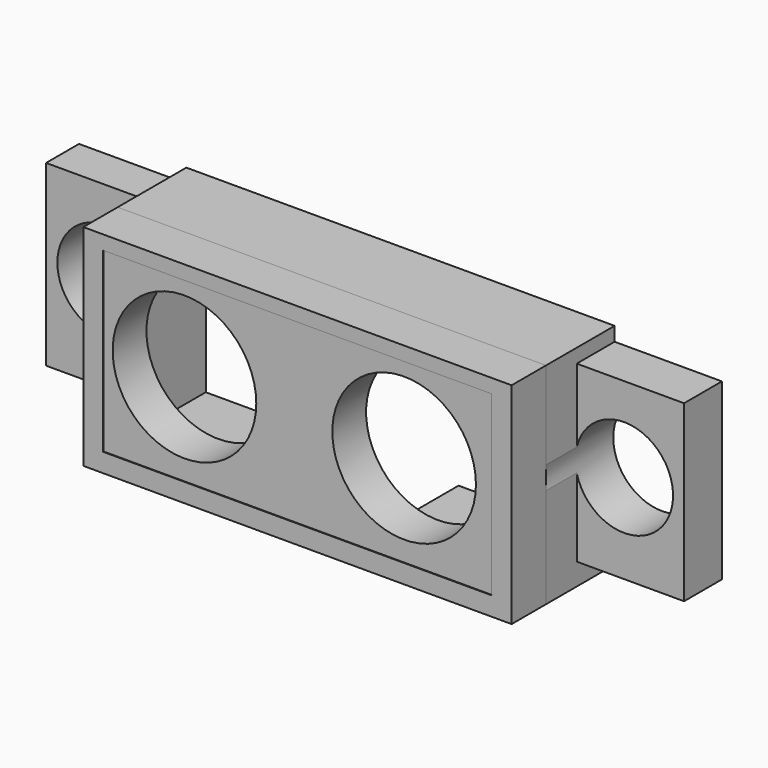
from build123d import *

# Parameters (mm, degrees)
F0_W      = 46
F0_H      = 21
F0_R      = 8.5
F1_DEPTH  = 5
F2_W      = 50.6975790486
F2_H      = 24.8879023129
F2_W_2    = 46
F2_H_2    = 21
F3_DEPTH  = 25.4
F4_W      = 14.5150721073
F4_H      = 25.4
F5_DEPTH  = 14.732
F6_W      = 50.6975790486
F6_H      = 24.8879023129
F7_DEPTH  = 10.16
F8_W      = 14.5150721073
F8_H      = 2.2287086546
F9_DEPTH  = 5.08
F10_DEPTH = 7.874
F12_W     = 2.0801138837
F12_H     = 21.1301185191
F14_DEPTH = 12.7
F13_W     = 2.8098069835
F13_H     = 20.6354465336
F15_DEPTH = 12.7
F16_DEPTH = 2.794
F17_R     = 5.7785
F18_DEPTH = 25.4


# Not quite as in the source:
# - a feature of the source that left no trace in its solid (it failed there, or was rolled back) is left out


with BuildPart() as f1:
    # F0 (on Front) → F1 (new body)
    with BuildSketch(Plane.XZ):
        with Locations((-23, -10.5)):
            Rectangle(F0_W, F0_H)
        with Locations((-36.3915145417, -10.1194066999)):
            Circle(F0_R, mode=Mode.SUBTRACT)
        with Locations((-10.3915145417, -10.1194066999)):
            Circle(F0_R, mode=Mode.SUBTRACT)
    extrude(amount=F1_DEPTH)


with BuildPart() as f3:
    # F2 (on face) → F3 (new body)
    with BuildSketch(Plane(origin=(0, 0, 0), x_dir=(-1, 0, 0), z_dir=(0, 1, 0))):
        with Locations((22.9521770962, -10.7847574982)):
            Rectangle(F2_W, F2_H)
        with Locations((23, -10.5)):
            Rectangle(F2_W_2, F2_H_2, mode=Mode.SUBTRACT)
    extrude(amount=F3_DEPTH)

    # F4 (on face) → F5 (cut)
    with BuildSketch(Plane.XY.offset(-21)):
        with Locations((-23.3345888555, 12.7)):
            Rectangle(F4_W, F4_H)
    extrude(amount=-F5_DEPTH, mode=Mode.SUBTRACT)

    # F6 (on face) → F7 (cut)
    with BuildSketch(Plane(origin=(0, 25.4, 0), x_dir=(-1, 0, 0), z_dir=(0, 1, 0))):
        with Locations((22.9521770962, -10.7847574982)):
            Rectangle(F6_W, F6_H)
    extrude(amount=-F7_DEPTH, mode=Mode.SUBTRACT)

    # F10 (cut): a face of the model
    f10_faces = [f3.faces().sort_by_distance(p)[0] for p in [
        (-47.7361965608, 15.24, -10.7847574982),
    ]]
    extrude(f10_faces, amount=-F10_DEPTH, mode=Mode.SUBTRACT)

    # F12 (on face) → F14 (join)
    with BuildSketch(Plane(origin=(-48.3009666204, 0, 0), x_dir=(0, -1, 0), z_dir=(-1, 0, 0))):
        with Locations((-6.3259430582, -10.5650592595)):
            Rectangle(F12_W, F12_H)
    extrude(amount=F14_DEPTH)

    # F13 (on face) → F15 (join)
    with BuildSketch(Plane.YZ.offset(2.3966124281)):
        with Locations((5.9610965082, -10.3177232668)):
            Rectangle(F13_W, F13_H)
    extrude(amount=F15_DEPTH)

    # F16 (add): a face of the model
    f16_faces = [f3.faces().sort_by_distance(p)[0] for p in [
        (-47.5003263005, 7.366, -22.1794135869),
    ]]
    extrude(f16_faces, amount=F16_DEPTH)

    # F17 (on face) → F18 (cut)
    with BuildSketch(Plane(origin=(0, 10.16, 0), x_dir=(-1, 0, 0), z_dir=(0, 1, 0))):
        with Locations((-8.016298525, -10.0460601971)):
            Circle(F17_R)
        with Locations((53.8871772587, -9.9512618035)):
            Circle(F17_R)
    extrude(amount=-F18_DEPTH, mode=Mode.SUBTRACT)


with BuildPart() as f9:
    # F8 (on face) → F9 (new body)
    with BuildSketch(Plane.XZ):
        Polygon((-48.3009666204, 1.6591936583), (-48.3009666204, -23.2287086546), (-30.5921249092, -23.2287086546), (-30.5921249092, -21), (-46, -21), (-46, 0), (0, 0), (0, -21), (-16.0770528018, -21), (-16.0770528018, -23.2287086546), (2.3966124281, -23.2287086546), (2.3966124281, 1.6591936583), align=None)
        with Locations((-23.3345888555, -22.1143543273)):
            Rectangle(F8_W, F8_H)
    extrude(amount=F9_DEPTH)


solid = Compound([f1.part, f3.part, f9.part])
